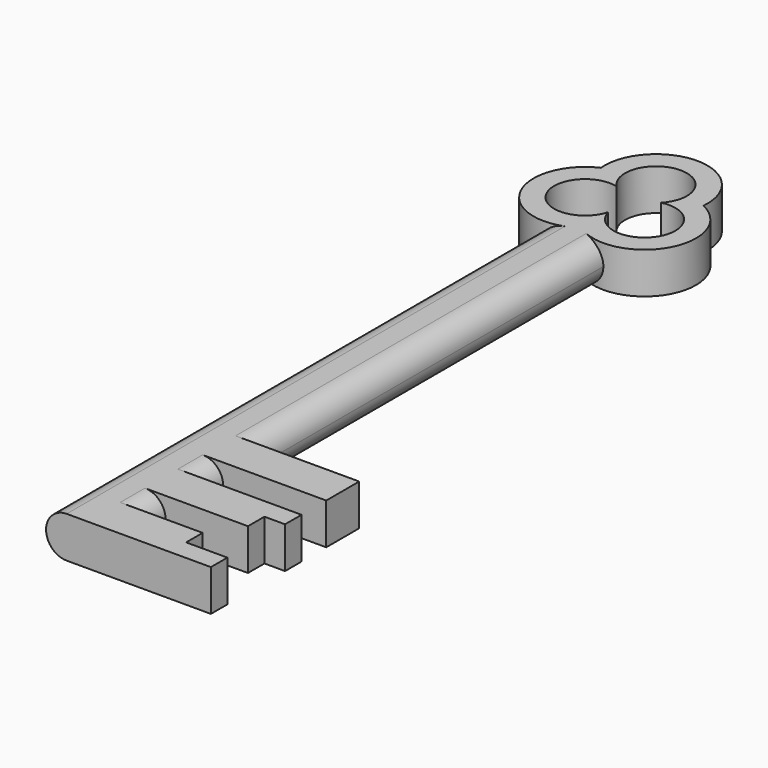
from build123d import *

# Parameters (mm, degrees)
F1_DEPTH = 50.8
F2_R     = 25.39999
F4_W     = 61.8233563619
F4_H     = 42.2021473569
F4_W_2   = 44.7444434271
F4_H_2   = 31.3514119965
F5_DEPTH = 50.8


# Not quite as in the source:
# - a fillet or chamfer is up to 0.001 mm smaller than in the source, because OpenCascade refuses the exact size


with BuildPart() as f1:
    # F0 (on Top) → F1 (new body)
    with BuildSketch(Plane.XY):
        with BuildLine():
            Line((-125.9584231198, 326.6096413136), (-125.9584231198, -437.0573322225))
            Line((-125.9584231198, -437.0573322225), (-49.7584231198, -437.0573322225))
            Line((-49.7584231198, -437.0573322225), (77.2415768802, -437.0573322225))
            Line((77.2415768802, -437.0573322225), (77.2415768802, -386.2573322225))
            Line((77.2415768802, -386.2573322225), (-49.7584231198, -386.2573322225))
            Line((-49.7584231198, -386.2573322225), (-49.7584231198, -348.1573322225))
            Line((-49.7584231198, -348.1573322225), (77.2415768802, -348.1573322225))
            Line((77.2415768802, -348.1573322225), (77.2415768802, -297.3573322225))
            Line((77.2415768802, -297.3573322225), (-49.7584231198, -297.3573322225))
            Line((-49.7584231198, -297.3573322225), (-49.7584231198, -259.2573322225))
            Line((-49.7584231198, -259.2573322225), (77.2415768802, -259.2573322225))
            Line((77.2415768802, -259.2573322225), (77.2415768802, -208.4573322225))
            Line((77.2415768802, -208.4573322225), (-49.7584231198, -208.4573322225))
            Line((-49.7584231198, -208.4573322225), (-49.7584231198, 326.6096413136))
            ThreePointArc((-49.7584231198, 326.6096413136), (12.201780711, 376.4463381022), (-23.1943939269, 447.6493859763))
            ThreePointArc((-23.1943939269, 447.6493859763), (-86.3855996742, 517.0444461389), (-149.6523168654, 447.718221991))
            ThreePointArc((-149.6523168654, 447.718221991), (-185.4004633868, 377.8523446501), (-125.9584231198, 326.6096413136))
        make_face()
        with BuildLine():
            ThreePointArc((-86.4201652133, 379.6749489688), (-156.0774751911, 370.9944555466), (-113.7312923812, 426.9792088355))
            ThreePointArc((-113.7312923812, 426.9792088355), (-86.4201652133, 491.6444555466), (-59.1090380455, 426.9792088355))
            ThreePointArc((-59.1090380455, 426.9792088355), (-16.7628552356, 370.9944555466), (-86.4201652133, 379.6749489688))
        make_face(mode=Mode.SUBTRACT)
    extrude(amount=F1_DEPTH)

    # F2 (radius 25.4 in the source; OpenCascade refuses exactly that, so slightly less here)
    f2_edges = [f1.edges().sort_by_distance(p)[0] for p in [
        (-125.958423, -55.223845, 50.8),
        (-49.758423, 59.076155, 50.8),
        (-49.758423, 59.076155, 0),
        (-125.958423, -55.223845, 0),
        (-49.758423, -278.307332, 0),
        (-49.758423, -367.207332, 0),
        (-49.758423, -367.207332, 50.8),
        (-49.758423, -278.307332, 50.8),
    ]]
    fillet(f2_edges, radius=F2_R)

    # F4 (on face) → F5 (cut)
    with BuildSketch(Plane.XY.offset(50.8)):
        with Locations((57.3532550612, -390.556258544)):
            Rectangle(F4_W, F4_H)
        with Locations((74.2137985938, -338.4330382207)):
            Rectangle(F4_W_2, F4_H_2)
    extrude(amount=-F5_DEPTH, mode=Mode.SUBTRACT)


solid = f1.part
